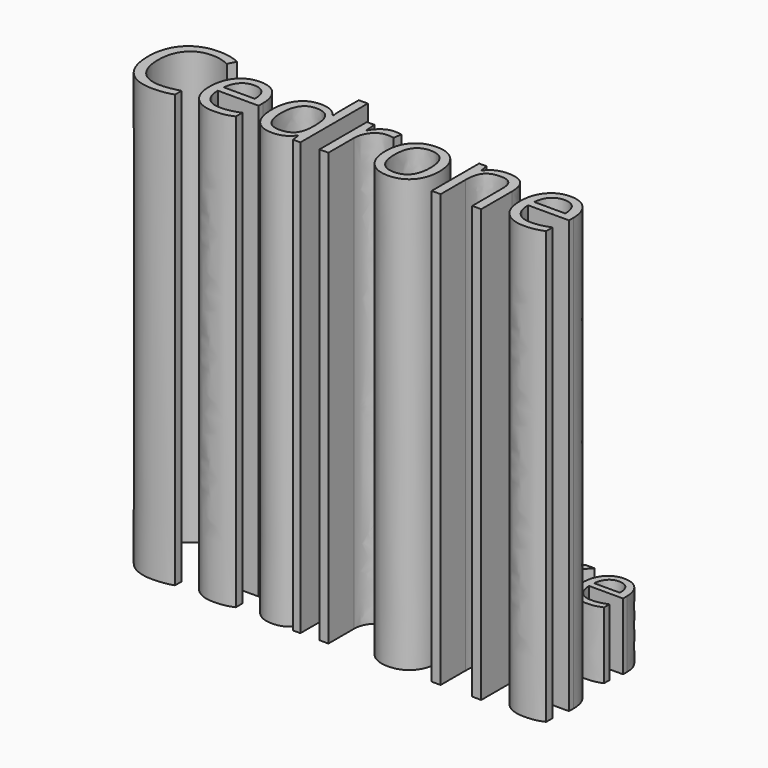
from build123d import *

# Parameters (mm, degrees)
F0_TEXT_SIZE = 87.5171687868
F1_DEPTH     = 63.5
F2_TEXT_SIZE = 105.3970307112
F3_DEPTH     = 410.8889698982


# Not quite as in the source:
# - Text() gives the source's letters only with a copy of the font that has no kerning and outlines rounded to 1/6400 em; it was checked with that copy


with BuildPart() as f1:
    # F0 (on Top) → F1 (new body)
    with BuildSketch(Plane.XY):
        with Locations((-175.0069884583, 0)):
            Text('Jake', F0_TEXT_SIZE, font='Open Sans', text_align=(TextAlign.LEFT, TextAlign.BOTTOM))
    extrude(amount=F1_DEPTH)


with BuildPart() as f3:
    # F2 (on Top) → F3 (new body)
    with BuildSketch(Plane.XY):
        with Locations((-422.0657031401, -75.885862112)):
            Text('Cedrone', F2_TEXT_SIZE, font='Open Sans', text_align=(TextAlign.LEFT, TextAlign.BOTTOM))
    extrude(amount=F3_DEPTH)


solid = Compound([f1.part, f3.part])
